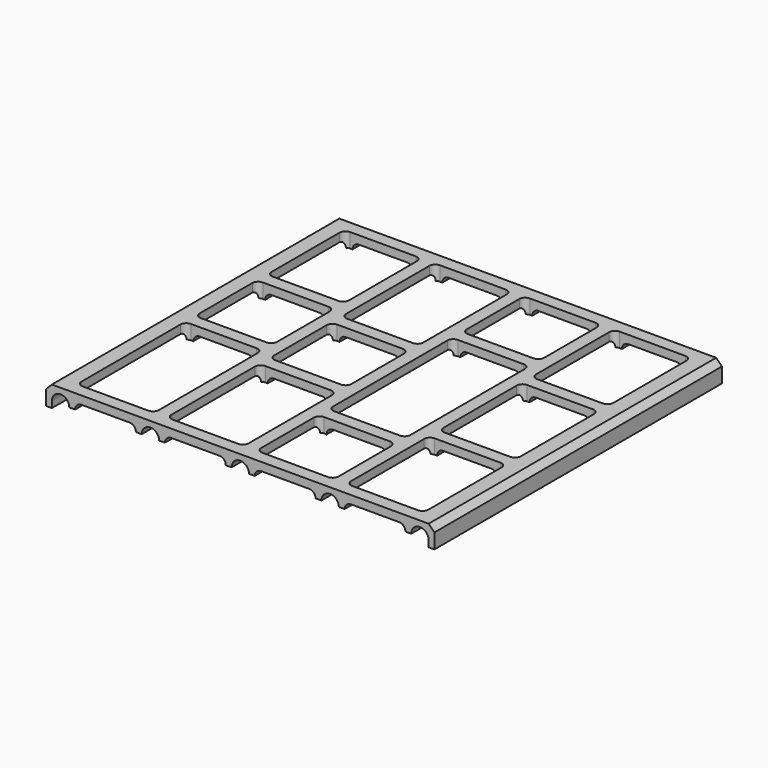
from build123d import *

# Parameters (mm, degrees)
F2_DEPTH      = 74.4
F3_R          = 1.29999
F4_SIZE       = 1.2
F6_W          = 16
F6_H          = 20
F6_H_2        = 16
F6_H_3        = 28
F6_H_4        = 24
F6_H_5        = 32
F6_H_6        = 21.3333333333
F7_DEPTH      = 1.701
F7_DEPTH_BACK = 2.601
F8_T4_DEPTH   = 4.7550100402
F8_S6_R       = 1.8
F8_T7_DEPTH   = 4
F8_T11_DEPTH  = 4.7550100402
F8_S12_R      = 1.8
F8_T13_DEPTH  = 4
F8_T18_DEPTH  = 4.7550100402
F8_S19_R      = 1.8
F8_T20_DEPTH  = 4
F8_T25_DEPTH  = 4.7550100402
F8_S26_R      = 1.8
F8_T27_DEPTH  = 4
F8_T32_DEPTH  = 4.7550100402
F8_S33_R      = 1.8
F8_T34_DEPTH  = 4
F8_T39_DEPTH  = 4.7550100402
F8_S40_R      = 1.8
F8_T41_DEPTH  = 4
F8_T46_DEPTH  = 4.7550100402
F8_S47_R      = 1.8
F8_T48_DEPTH  = 4
F8_T53_DEPTH  = 4.7550100402
F8_S54_R      = 1.8
F8_T55_DEPTH  = 4
F8_T60_DEPTH  = 4.7550100402
F8_S61_R      = 1.8
F8_T62_DEPTH  = 4
F8_T67_DEPTH  = 4.7550100402
F8_S68_R      = 1.8
F8_T69_DEPTH  = 4
F8_T74_DEPTH  = 4.7550100402
F8_S75_R      = 1.8
F8_T76_DEPTH  = 4
F8_T81_DEPTH  = 4.7550100402
F8_S82_R      = 1.8
F8_T83_DEPTH  = 4
F8_T88_DEPTH  = 4.7550100402
F8_S89_R      = 1.8
F8_T90_DEPTH  = 4
F8_T95_DEPTH  = 4.7550100402
F8_S96_R      = 1.8
F8_T97_DEPTH  = 4
F8_T102_DEPTH = 4.7550100402
F8_S103_R     = 1.8
F8_T104_DEPTH = 4
F8_T109_DEPTH = 4.7550100402
F8_S110_R     = 1.8
F8_T111_DEPTH = 4
F8_T116_DEPTH = 4.7550100402
F8_S117_R     = 1.8
F8_T118_DEPTH = 4
F8_T123_DEPTH = 4.7550100402
F8_S125_R     = 1.8
F8_T126_DEPTH = 4
F8_T130_DEPTH = 4.7550100402
F8_S131_R     = 1.8
F8_T132_DEPTH = 4
F8_T137_DEPTH = 4.7550100402
F8_S138_R     = 1.8
F8_T139_DEPTH = 4
F8_T144_DEPTH = 4.7550100402
F8_S145_R     = 1.8
F8_T146_DEPTH = 4
F8_T151_DEPTH = 4.7550100402
F8_S152_R     = 1.8
F8_T153_DEPTH = 4
F8_T158_DEPTH = 4.7550100402
F8_S159_R     = 1.8
F8_T160_DEPTH = 4
F8_T165_DEPTH = 4.7550100402
F8_S166_R     = 1.8
F8_T167_DEPTH = 4
F8_T172_DEPTH = 4.7550100402
F8_S173_R     = 1.8
F8_T174_DEPTH = 4
F8_T179_DEPTH = 4.7550100402
F8_S180_R     = 1.8
F8_T181_DEPTH = 4
F8_T186_DEPTH = 4.7550100402
F8_S187_R     = 1.8
F8_T188_DEPTH = 4
F8_T193_DEPTH = 4.7550100402
F8_S194_R     = 1.8
F8_T195_DEPTH = 4
F8_T200_DEPTH = 4.7550100402
F8_S201_R     = 1.8
F8_T202_DEPTH = 4
F8_T207_DEPTH = 4.7550100402
F8_S209_R     = 1.8
F8_T210_DEPTH = 4
F8_T214_DEPTH = 4.7550100402
F8_S216_R     = 1.8
F8_T217_DEPTH = 4
F8_T221_DEPTH = 4.7550100402
F8_S222_R     = 1.8
F8_T223_DEPTH = 4
F8_T228_DEPTH = 4.7550100402
F8_S229_R     = 1.8
F8_T230_DEPTH = 4
F8_T235_DEPTH = 4.7550100402
F8_S236_R     = 1.8
F8_T237_DEPTH = 4
F8_T242_DEPTH = 4.7550100402
F8_S243_R     = 1.8
F8_T244_DEPTH = 4
F8_T249_DEPTH = 4.7550100402
F8_S250_R     = 1.8
F8_T251_DEPTH = 4
F8_T256_DEPTH = 4.7550100402
F8_S257_R     = 1.8
F8_T258_DEPTH = 4
F8_T263_DEPTH = 4.7550100402
F8_S264_R     = 1.8
F8_T265_DEPTH = 4
F8_T270_DEPTH = 4.7550100402
F8_S271_R     = 1.8
F8_T272_DEPTH = 4
F8_T277_DEPTH = 4.7550100402
F8_S278_R     = 1.8
F8_T279_DEPTH = 4
F8_T284_DEPTH = 4.7550100402
F8_S285_R     = 1.8
F8_T286_DEPTH = 4
F8_T291_DEPTH = 4.7550100402
F8_S292_R     = 1.8
F8_T293_DEPTH = 4
F8_T298_DEPTH = 4.7550100402
F8_S299_R     = 1.8
F8_T300_DEPTH = 4
F8_T305_DEPTH = 4.7550100402
F8_S306_R     = 1.8
F8_T307_DEPTH = 4
F8_T312_DEPTH = 4.7550100402
F8_S313_R     = 1.8
F8_T314_DEPTH = 4
F8_T319_DEPTH = 4.7550100402
F8_S320_R     = 1.8
F8_T321_DEPTH = 4
F8_T326_DEPTH = 4.7550100402
F8_S327_R     = 1.8
F8_T328_DEPTH = 4
F8_T333_DEPTH = 4.7550100402
F8_S334_R     = 1.8
F8_T335_DEPTH = 4


# Not quite as in the source:
# - a fillet or chamfer that OpenCascade refuses, or shapes differently, is made with other operations: its cross-section is extruded or revolved along the edge and cut away or added
# - a fillet or chamfer is up to 0.001 mm smaller than in the source, because OpenCascade refuses the exact size


with BuildPart() as f2:
    # F1 (on Front) → F2 (new body)
    with BuildSketch(Plane.XZ):
        with BuildLine():
            ThreePointArc((-39, -1.3), (-37.2, 0.5), (-35.4, -1.3))
            Line((-35.4, -1.3), (-34.2, -1.3))
            Line((-34.2, -1.3), (-34.2, 0))
            Line((-34.2, 0), (-21.6, 0))
            Line((-21.6, 0), (-21.6, -1.3))
            Line((-21.6, -1.3), (-20.4, -1.3))
            ThreePointArc((-20.4, -1.3), (-18.6, 0.5), (-16.8, -1.3))
            Line((-16.8, -1.3), (-15.6, -1.3))
            Line((-15.6, -1.3), (-15.6, 0))
            Line((-15.6, 0), (-3, 0))
            Line((-3, 0), (-3, -1.3))
            Line((-3, -1.3), (-1.8, -1.3))
            ThreePointArc((-1.8, -1.3), (-1.2727922061, -0.0272077939), (0, 0.5))
            Line((0, 0.5), (0, 1.7))
            Line((0, 1.7), (-40.2, 1.7))
            Line((-40.2, 1.7), (-40.2, -2.6))
            Line((-40.2, -2.6), (-39, -2.6))
            Line((-39, -2.6), (-39, -1.3))
        make_face()
    extrude(amount=F2_DEPTH)

    # F3 (radius 1.3 in the source; OpenCascade refuses exactly that, so slightly less here)
    f3_edges = [f2.edges().sort_by_distance(p)[0] for p in [
        (-34.2, -37.2, 0),
        (-21.6, -37.2, 0),
        (-15.6, -37.2, 0),
        (-3, -37.2, 0),
    ]]
    fillet(f3_edges, radius=F3_R)

    # F4
    f4_edges = [f2.edges().sort_by_distance(p)[0] for p in [
        (-40.2, -37.2, 1.7),
    ]]
    chamfer(f4_edges, length=F4_SIZE)

    # F5: F2 across plane


with BuildPart() as f2_1:
    add(f2.part)
    add(f2.part.mirror(Plane.YZ))

    # F6 (on Top) → F7 (cut, two sides)
    with BuildSketch(Plane.XY) as f7_sk:
        with Locations((-27.9, -12.6)):
            Rectangle(F6_W, F6_H)
        with Locations((-27.9, -33.2)):
            Rectangle(F6_W, F6_H_2)
        with Locations((-27.9, -57.8)):
            Rectangle(F6_W, F6_H_3)
        with Locations((-9.3, -59.8)):
            Rectangle(F6_W, F6_H_4)
        with Locations((9.3, -63.8)):
            Rectangle(F6_W, F6_H_2)
        with Locations((-9.3, -37.2)):
            Rectangle(F6_W, F6_H_2)
        with Locations((-9.3, -14.6)):
            Rectangle(F6_W, F6_H_4)
        with Locations((9.3, -10.6)):
            Rectangle(F6_W, F6_H_2)
        with Locations((9.3, -37.2)):
            Rectangle(F6_W, F6_H_5)
        with Locations((27.9, -13.2666666667)):
            Rectangle(F6_W, F6_H_6)
        with Locations((27.9, -61.1333333333)):
            Rectangle(F6_W, F6_H_6)
        with Locations((27.9, -37.2)):
            Rectangle(F6_W, F6_H_6)
    extrude(amount=F7_DEPTH, mode=Mode.SUBTRACT)
    extrude(f7_sk.sketch, amount=-F7_DEPTH_BACK, mode=Mode.SUBTRACT)

    # F8: fillet of radius 1.2 on 48 edges, made by hand


with BuildPart() as f8_tool2:
    # F8_s3 → F8_t4 (new body)
    with BuildSketch(Plane.XY.offset(1.7)):
        with BuildLine():
            ThreePointArc((-21.1, -2.6), (-20.2514718626, -2.9514718626), (-19.9, -3.8))
            Line((-19.9, -3.8), (-19.9, -2.6))
            Line((-19.9, -2.6), (-21.1, -2.6))
        make_face()
    extrude(amount=-F8_T4_DEPTH)

    split(bisect_by=Plane.XY.offset(-1.3), keep=Keep.TOP)

    # F8_s6 → F8_t7 (cut, symmetric)
    with BuildSketch(Plane.XZ.offset(3.2)):
        with Locations((-18.6, -1.3)):
            Circle(F8_S6_R)
    extrude(amount=F8_T7_DEPTH, both=True, mode=Mode.SUBTRACT)


with BuildPart() as f2_2:
    add(f2_1.part)

    # F8_t1: union F8_tool2
    add(f8_tool2.part)


with BuildPart() as f8_tool9:
    # F8_s10 → F8_t11 (new body)
    with BuildSketch(Plane.XY.offset(-3.0550100402)):
        with BuildLine():
            ThreePointArc((-34.7, -2.6), (-35.5485281374, -2.9514718626), (-35.9, -3.8))
            Line((-35.9, -3.8), (-35.9, -2.6))
            Line((-35.9, -2.6), (-34.7, -2.6))
        make_face()
    extrude(amount=F8_T11_DEPTH)

    # F8_s12 → F8_t13 (cut, symmetric)
    with BuildSketch(Plane.XZ.offset(3.2)):
        with Locations((-37.2, -1.3)):
            Circle(F8_S12_R)
    extrude(amount=F8_T13_DEPTH, both=True, mode=Mode.SUBTRACT)

    split(bisect_by=Plane.XY.offset(-1.3), keep=Keep.TOP)


with BuildPart() as f2_3:
    add(f2_2.part)

    # F8_t8: union F8_tool9
    add(f8_tool9.part)


with BuildPart() as f8_tool16:
    # F8_s17 → F8_t18 (new body)
    with BuildSketch(Plane.XY.offset(1.7)):
        with BuildLine():
            ThreePointArc((-21.1, -22.6), (-20.2514718626, -22.2485281374), (-19.9, -21.4))
            Line((-19.9, -21.4), (-19.9, -22.6))
            Line((-19.9, -22.6), (-21.1, -22.6))
        make_face()
    extrude(amount=-F8_T18_DEPTH)

    # F8_s19 → F8_t20 (cut, symmetric)
    with BuildSketch(Plane.XZ.offset(22)):
        with Locations((-18.6, -1.3)):
            Circle(F8_S19_R)
    extrude(amount=F8_T20_DEPTH, both=True, mode=Mode.SUBTRACT)

    split(bisect_by=Plane.XY.offset(-1.3), keep=Keep.TOP)


with BuildPart() as f2_4:
    add(f2_3.part)

    # F8_t15: union F8_tool16
    add(f8_tool16.part)


with BuildPart() as f8_tool23:
    # F8_s24 → F8_t25 (new body)
    with BuildSketch(Plane.XY.offset(-3.0550100402)):
        with BuildLine():
            ThreePointArc((-35.9, -21.4), (-35.5485281374, -22.2485281374), (-34.7, -22.6))
            Line((-34.7, -22.6), (-35.9, -22.6))
            Line((-35.9, -22.6), (-35.9, -21.4))
        make_face()
    extrude(amount=F8_T25_DEPTH)

    # F8_s26 → F8_t27 (cut, symmetric)
    with BuildSketch(Plane.XZ.offset(22)):
        with Locations((-37.2, -1.3)):
            Circle(F8_S26_R)
    extrude(amount=F8_T27_DEPTH, both=True, mode=Mode.SUBTRACT)

    split(bisect_by=Plane.XY.offset(-1.3), keep=Keep.TOP)


with BuildPart() as f2_5:
    add(f2_4.part)

    # F8_t22: union F8_tool23
    add(f8_tool23.part)


with BuildPart() as f8_tool30:
    # F8_s31 → F8_t32 (new body)
    with BuildSketch(Plane.XY.offset(-3.0550100402)):
        with BuildLine():
            ThreePointArc((-34.7, -25.2), (-35.5485281374, -25.5514718626), (-35.9, -26.4))
            Line((-35.9, -26.4), (-35.9, -25.2))
            Line((-35.9, -25.2), (-34.7, -25.2))
        make_face()
    extrude(amount=F8_T32_DEPTH)

    # F8_s33 → F8_t34 (cut, symmetric)
    with BuildSketch(Plane.XZ.offset(25.8)):
        with Locations((-37.2, -1.3)):
            Circle(F8_S33_R)
    extrude(amount=F8_T34_DEPTH, both=True, mode=Mode.SUBTRACT)

    split(bisect_by=Plane.XY.offset(-1.3), keep=Keep.TOP)


with BuildPart() as f2_6:
    add(f2_5.part)

    # F8_t29: union F8_tool30
    add(f8_tool30.part)


with BuildPart() as f8_tool37:
    # F8_s38 → F8_t39 (new body)
    with BuildSketch(Plane.XY.offset(-3.0550100402)):
        with BuildLine():
            ThreePointArc((-35.9, -40), (-35.5485281374, -40.8485281374), (-34.7, -41.2))
            Line((-34.7, -41.2), (-35.9, -41.2))
            Line((-35.9, -41.2), (-35.9, -40))
        make_face()
    extrude(amount=F8_T39_DEPTH)

    # F8_s40 → F8_t41 (cut, symmetric)
    with BuildSketch(Plane.XZ.offset(40.6)):
        with Locations((-37.2, -1.3)):
            Circle(F8_S40_R)
    extrude(amount=F8_T41_DEPTH, both=True, mode=Mode.SUBTRACT)

    split(bisect_by=Plane.XY.offset(-1.3), keep=Keep.TOP)


with BuildPart() as f2_7:
    add(f2_6.part)

    # F8_t36: union F8_tool37
    add(f8_tool37.part)


with BuildPart() as f8_tool44:
    # F8_s45 → F8_t46 (new body)
    with BuildSketch(Plane.XY.offset(-3.0550100402)):
        with BuildLine():
            ThreePointArc((-35.9, -70.6), (-35.5485281374, -71.4485281374), (-34.7, -71.8))
            Line((-34.7, -71.8), (-35.9, -71.8))
            Line((-35.9, -71.8), (-35.9, -70.6))
        make_face()
    extrude(amount=F8_T46_DEPTH)

    # F8_s47 → F8_t48 (cut, symmetric)
    with BuildSketch(Plane.XZ.offset(71.2)):
        with Locations((-37.2, -1.3)):
            Circle(F8_S47_R)
    extrude(amount=F8_T48_DEPTH, both=True, mode=Mode.SUBTRACT)

    split(bisect_by=Plane.XY.offset(-1.3), keep=Keep.TOP)


with BuildPart() as f2_8:
    add(f2_7.part)

    # F8_t43: union F8_tool44
    add(f8_tool44.part)


with BuildPart() as f8_tool51:
    # F8_s52 → F8_t53 (new body)
    with BuildSketch(Plane.XY.offset(-3.0550100402)):
        with BuildLine():
            ThreePointArc((-34.7, -43.8), (-35.5485281374, -44.1514718626), (-35.9, -45))
            Line((-35.9, -45), (-35.9, -43.8))
            Line((-35.9, -43.8), (-34.7, -43.8))
        make_face()
    extrude(amount=F8_T53_DEPTH)

    # F8_s54 → F8_t55 (cut, symmetric)
    with BuildSketch(Plane.XZ.offset(44.4)):
        with Locations((-37.2, -1.3)):
            Circle(F8_S54_R)
    extrude(amount=F8_T55_DEPTH, both=True, mode=Mode.SUBTRACT)

    split(bisect_by=Plane.XY.offset(-1.3), keep=Keep.TOP)


with BuildPart() as f2_9:
    add(f2_8.part)

    # F8_t50: union F8_tool51
    add(f8_tool51.part)


with BuildPart() as f8_tool58:
    # F8_s59 → F8_t60 (new body)
    with BuildSketch(Plane.XY.offset(1.7)):
        with BuildLine():
            ThreePointArc((-21.1, -25.2), (-20.2514718626, -25.5514718626), (-19.9, -26.4))
            Line((-19.9, -26.4), (-19.9, -25.2))
            Line((-19.9, -25.2), (-21.1, -25.2))
        make_face()
    extrude(amount=-F8_T60_DEPTH)

    # F8_s61 → F8_t62 (cut, symmetric)
    with BuildSketch(Plane.XZ.offset(25.8)):
        with Locations((-18.6, -1.3)):
            Circle(F8_S61_R)
    extrude(amount=F8_T62_DEPTH, both=True, mode=Mode.SUBTRACT)

    split(bisect_by=Plane.XY.offset(-1.3), keep=Keep.TOP)


with BuildPart() as f2_10:
    add(f2_9.part)

    # F8_t57: union F8_tool58
    add(f8_tool58.part)


with BuildPart() as f8_tool65:
    # F8_s66 → F8_t67 (new body)
    with BuildSketch(Plane.XY.offset(1.7)):
        with BuildLine():
            ThreePointArc((-21.1, -41.2), (-20.2514718626, -40.8485281374), (-19.9, -40))
            Line((-19.9, -40), (-19.9, -41.2))
            Line((-19.9, -41.2), (-21.1, -41.2))
        make_face()
    extrude(amount=-F8_T67_DEPTH)

    # F8_s68 → F8_t69 (cut, symmetric)
    with BuildSketch(Plane.XZ.offset(40.6)):
        with Locations((-18.6, -1.3)):
            Circle(F8_S68_R)
    extrude(amount=F8_T69_DEPTH, both=True, mode=Mode.SUBTRACT)

    split(bisect_by=Plane.XY.offset(-1.3), keep=Keep.TOP)


with BuildPart() as f2_11:
    add(f2_10.part)

    # F8_t64: union F8_tool65
    add(f8_tool65.part)


with BuildPart() as f8_tool72:
    # F8_s73 → F8_t74 (new body)
    with BuildSketch(Plane.XY.offset(1.7)):
        with BuildLine():
            ThreePointArc((-21.1, -43.8), (-20.2514718626, -44.1514718626), (-19.9, -45))
            Line((-19.9, -45), (-19.9, -43.8))
            Line((-19.9, -43.8), (-21.1, -43.8))
        make_face()
    extrude(amount=-F8_T74_DEPTH)

    # F8_s75 → F8_t76 (cut, symmetric)
    with BuildSketch(Plane.XZ.offset(44.4)):
        with Locations((-18.6, -1.3)):
            Circle(F8_S75_R)
    extrude(amount=F8_T76_DEPTH, both=True, mode=Mode.SUBTRACT)

    split(bisect_by=Plane.XY.offset(-1.3), keep=Keep.TOP)


with BuildPart() as f2_12:
    add(f2_11.part)

    # F8_t71: union F8_tool72
    add(f8_tool72.part)


with BuildPart() as f8_tool79:
    # F8_s80 → F8_t81 (new body)
    with BuildSketch(Plane.XY.offset(1.7)):
        with BuildLine():
            ThreePointArc((-21.1, -71.8), (-20.2514718626, -71.4485281374), (-19.9, -70.6))
            Line((-19.9, -70.6), (-19.9, -71.8))
            Line((-19.9, -71.8), (-21.1, -71.8))
        make_face()
    extrude(amount=-F8_T81_DEPTH)

    # F8_s82 → F8_t83 (cut, symmetric)
    with BuildSketch(Plane.XZ.offset(71.2)):
        with Locations((-18.6, -1.3)):
            Circle(F8_S82_R)
    extrude(amount=F8_T83_DEPTH, both=True, mode=Mode.SUBTRACT)

    split(bisect_by=Plane.XY.offset(-1.3), keep=Keep.TOP)


with BuildPart() as f2_13:
    add(f2_12.part)

    # F8_t78: union F8_tool79
    add(f8_tool79.part)


with BuildPart() as f8_tool86:
    # F8_s87 → F8_t88 (new body)
    with BuildSketch(Plane.XY.offset(-3.0550100402)):
        with BuildLine():
            ThreePointArc((-17.3, -25.4), (-16.9485281374, -26.2485281374), (-16.1, -26.6))
            Line((-16.1, -26.6), (-17.3, -26.6))
            Line((-17.3, -26.6), (-17.3, -25.4))
        make_face()
    extrude(amount=F8_T88_DEPTH)

    # F8_s89 → F8_t90 (cut, symmetric)
    with BuildSketch(Plane.XZ.offset(26)):
        with Locations((-18.6, -1.3)):
            Circle(F8_S89_R)
    extrude(amount=F8_T90_DEPTH, both=True, mode=Mode.SUBTRACT)

    split(bisect_by=Plane.XY.offset(-1.3), keep=Keep.TOP)


with BuildPart() as f2_14:
    add(f2_13.part)

    # F8_t85: union F8_tool86
    add(f8_tool86.part)


with BuildPart() as f8_tool93:
    # F8_s94 → F8_t95 (new body)
    with BuildSketch(Plane.XY.offset(-3.0550100402)):
        with BuildLine():
            ThreePointArc((-17.3, -44), (-16.9485281374, -44.8485281374), (-16.1, -45.2))
            Line((-16.1, -45.2), (-17.3, -45.2))
            Line((-17.3, -45.2), (-17.3, -44))
        make_face()
    extrude(amount=F8_T95_DEPTH)

    # F8_s96 → F8_t97 (cut, symmetric)
    with BuildSketch(Plane.XZ.offset(44.6)):
        with Locations((-18.6, -1.3)):
            Circle(F8_S96_R)
    extrude(amount=F8_T97_DEPTH, both=True, mode=Mode.SUBTRACT)

    split(bisect_by=Plane.XY.offset(-1.3), keep=Keep.TOP)


with BuildPart() as f2_15:
    add(f2_14.part)

    # F8_t92: union F8_tool93
    add(f8_tool93.part)


with BuildPart() as f8_tool100:
    # F8_s101 → F8_t102 (new body)
    with BuildSketch(Plane.XY.offset(-3.0550100402)):
        with BuildLine():
            ThreePointArc((-17.3, -70.6), (-16.9485281374, -71.4485281374), (-16.1, -71.8))
            Line((-16.1, -71.8), (-17.3, -71.8))
            Line((-17.3, -71.8), (-17.3, -70.6))
        make_face()
    extrude(amount=F8_T102_DEPTH)

    # F8_s103 → F8_t104 (cut, symmetric)
    with BuildSketch(Plane.XZ.offset(71.2)):
        with Locations((-18.6, -1.3)):
            Circle(F8_S103_R)
    extrude(amount=F8_T104_DEPTH, both=True, mode=Mode.SUBTRACT)

    split(bisect_by=Plane.XY.offset(-1.3), keep=Keep.TOP)


with BuildPart() as f2_16:
    add(f2_15.part)

    # F8_t99: union F8_tool100
    add(f8_tool100.part)


with BuildPart() as f8_tool107:
    # F8_s108 → F8_t109 (new body)
    with BuildSketch(Plane.XY.offset(-3.0550100402)):
        with BuildLine():
            ThreePointArc((-16.1, -2.6), (-16.9485281374, -2.9514718626), (-17.3, -3.8))
            Line((-17.3, -3.8), (-17.3, -2.6))
            Line((-17.3, -2.6), (-16.1, -2.6))
        make_face()
    extrude(amount=F8_T109_DEPTH)

    # F8_s110 → F8_t111 (cut, symmetric)
    with BuildSketch(Plane.XZ.offset(3.2)):
        with Locations((-18.6, -1.3)):
            Circle(F8_S110_R)
    extrude(amount=F8_T111_DEPTH, both=True, mode=Mode.SUBTRACT)

    split(bisect_by=Plane.XY.offset(-1.3), keep=Keep.TOP)


with BuildPart() as f2_17:
    add(f2_16.part)

    # F8_t106: union F8_tool107
    add(f8_tool107.part)


with BuildPart() as f8_tool114:
    # F8_s115 → F8_t116 (new body)
    with BuildSketch(Plane.XY.offset(-3.0550100402)):
        with BuildLine():
            ThreePointArc((-16.1, -29.2), (-16.9485281374, -29.5514718626), (-17.3, -30.4))
            Line((-17.3, -30.4), (-17.3, -29.2))
            Line((-17.3, -29.2), (-16.1, -29.2))
        make_face()
    extrude(amount=F8_T116_DEPTH)

    # F8_s117 → F8_t118 (cut, symmetric)
    with BuildSketch(Plane.XZ.offset(29.8)):
        with Locations((-18.6, -1.3)):
            Circle(F8_S117_R)
    extrude(amount=F8_T118_DEPTH, both=True, mode=Mode.SUBTRACT)

    split(bisect_by=Plane.XY.offset(-1.3), keep=Keep.TOP)


with BuildPart() as f2_18:
    add(f2_17.part)

    # F8_t113: union F8_tool114
    add(f8_tool114.part)


with BuildPart() as f8_tool121:
    # F8_s122 → F8_t123 (new body)
    with BuildSketch(Plane.XY.offset(1.7)):
        with BuildLine():
            ThreePointArc((-2.5, -2.6), (-1.6514718626, -2.9514718626), (-1.3, -3.8))
            Line((-1.3, -3.8), (-1.3, -2.6))
            Line((-1.3, -2.6), (-2.5, -2.6))
        make_face()
    extrude(amount=-F8_T123_DEPTH)

    split(bisect_by=Plane.XY.offset(-1.3), keep=Keep.TOP)

    # F8_s125 → F8_t126 (cut, symmetric)
    with BuildSketch(Plane.XZ.offset(3.2)):
        with Locations((0, -1.3)):
            Circle(F8_S125_R)
    extrude(amount=F8_T126_DEPTH, both=True, mode=Mode.SUBTRACT)


with BuildPart() as f2_19:
    add(f2_18.part)

    # F8_t120: union F8_tool121
    add(f8_tool121.part)


with BuildPart() as f8_tool128:
    # F8_s129 → F8_t130 (new body)
    with BuildSketch(Plane.XY.offset(1.7)):
        with BuildLine():
            ThreePointArc((-2.5, -29.2), (-1.6514718626, -29.5514718626), (-1.3, -30.4))
            Line((-1.3, -30.4), (-1.3, -29.2))
            Line((-1.3, -29.2), (-2.5, -29.2))
        make_face()
    extrude(amount=-F8_T130_DEPTH)

    # F8_s131 → F8_t132 (cut, symmetric)
    with BuildSketch(Plane.XZ.offset(29.8)):
        with Locations((0, -1.3)):
            Circle(F8_S131_R)
    extrude(amount=F8_T132_DEPTH, both=True, mode=Mode.SUBTRACT)

    split(bisect_by=Plane.XY.offset(-1.3), keep=Keep.TOP)


with BuildPart() as f2_20:
    add(f2_19.part)

    # F8_t127: union F8_tool128
    add(f8_tool128.part)


with BuildPart() as f8_tool135:
    # F8_s136 → F8_t137 (new body)
    with BuildSketch(Plane.XY.offset(1.7)):
        with BuildLine():
            ThreePointArc((-2.5, -47.8), (-1.6514718626, -48.1514718626), (-1.3, -49))
            Line((-1.3, -49), (-1.3, -47.8))
            Line((-1.3, -47.8), (-2.5, -47.8))
        make_face()
    extrude(amount=-F8_T137_DEPTH)

    # F8_s138 → F8_t139 (cut, symmetric)
    with BuildSketch(Plane.XZ.offset(48.4)):
        with Locations((0, -1.3)):
            Circle(F8_S138_R)
    extrude(amount=F8_T139_DEPTH, both=True, mode=Mode.SUBTRACT)

    split(bisect_by=Plane.XY.offset(-1.3), keep=Keep.TOP)


with BuildPart() as f2_21:
    add(f2_20.part)

    # F8_t134: union F8_tool135
    add(f8_tool135.part)


with BuildPart() as f8_tool142:
    # F8_s143 → F8_t144 (new body)
    with BuildSketch(Plane.XY.offset(1.7)):
        with BuildLine():
            ThreePointArc((-2.5, -71.8), (-1.6514718626, -71.4485281374), (-1.3, -70.6))
            Line((-1.3, -70.6), (-1.3, -71.8))
            Line((-1.3, -71.8), (-2.5, -71.8))
        make_face()
    extrude(amount=-F8_T144_DEPTH)

    # F8_s145 → F8_t146 (cut, symmetric)
    with BuildSketch(Plane.XZ.offset(71.2)):
        with Locations((0, -1.3)):
            Circle(F8_S145_R)
    extrude(amount=F8_T146_DEPTH, both=True, mode=Mode.SUBTRACT)

    split(bisect_by=Plane.XY.offset(-1.3), keep=Keep.TOP)


with BuildPart() as f2_22:
    add(f2_21.part)

    # F8_t141: union F8_tool142
    add(f8_tool142.part)


with BuildPart() as f8_tool149:
    # F8_s150 → F8_t151 (new body)
    with BuildSketch(Plane.XY.offset(1.7)):
        with BuildLine():
            ThreePointArc((-2.5, -45.2), (-1.6514718626, -44.8485281374), (-1.3, -44))
            Line((-1.3, -44), (-1.3, -45.2))
            Line((-1.3, -45.2), (-2.5, -45.2))
        make_face()
    extrude(amount=-F8_T151_DEPTH)

    # F8_s152 → F8_t153 (cut, symmetric)
    with BuildSketch(Plane.XZ.offset(44.6)):
        with Locations((0, -1.3)):
            Circle(F8_S152_R)
    extrude(amount=F8_T153_DEPTH, both=True, mode=Mode.SUBTRACT)

    split(bisect_by=Plane.XY.offset(-1.3), keep=Keep.TOP)


with BuildPart() as f2_23:
    add(f2_22.part)

    # F8_t148: union F8_tool149
    add(f8_tool149.part)


with BuildPart() as f8_tool156:
    # F8_s157 → F8_t158 (new body)
    with BuildSketch(Plane.XY.offset(1.7)):
        with BuildLine():
            ThreePointArc((-2.5, -26.6), (-1.6514718626, -26.2485281374), (-1.3, -25.4))
            Line((-1.3, -25.4), (-1.3, -26.6))
            Line((-1.3, -26.6), (-2.5, -26.6))
        make_face()
    extrude(amount=-F8_T158_DEPTH)

    # F8_s159 → F8_t160 (cut, symmetric)
    with BuildSketch(Plane.XZ.offset(26)):
        with Locations((0, -1.3)):
            Circle(F8_S159_R)
    extrude(amount=F8_T160_DEPTH, both=True, mode=Mode.SUBTRACT)

    split(bisect_by=Plane.XY.offset(-1.3), keep=Keep.TOP)


with BuildPart() as f2_24:
    add(f2_23.part)

    # F8_t155: union F8_tool156
    add(f8_tool156.part)


with BuildPart() as f8_tool163:
    # F8_s164 → F8_t165 (new body)
    with BuildSketch(Plane.XY.offset(-3.0550100402)):
        with BuildLine():
            ThreePointArc((16.1, -71.8), (16.9485281374, -71.4485281374), (17.3, -70.6))
            Line((17.3, -70.6), (17.3, -71.8))
            Line((17.3, -71.8), (16.1, -71.8))
        make_face()
    extrude(amount=F8_T165_DEPTH)

    # F8_s166 → F8_t167 (cut, symmetric)
    with BuildSketch(Plane.XZ.offset(71.2)):
        with Locations((18.6, -1.3)):
            Circle(F8_S166_R)
    extrude(amount=F8_T167_DEPTH, both=True, mode=Mode.SUBTRACT)

    split(bisect_by=Plane.XY.offset(-1.3), keep=Keep.TOP)


with BuildPart() as f2_25:
    add(f2_24.part)

    # F8_t162: union F8_tool163
    add(f8_tool163.part)


with BuildPart() as f8_tool170:
    # F8_s171 → F8_t172 (new body)
    with BuildSketch(Plane.XY.offset(1.7)):
        with BuildLine():
            ThreePointArc((16.1, -53.2), (16.9485281374, -52.8485281374), (17.3, -52))
            Line((17.3, -52), (17.3, -53.2))
            Line((17.3, -53.2), (16.1, -53.2))
        make_face()
    extrude(amount=-F8_T172_DEPTH)

    # F8_s173 → F8_t174 (cut, symmetric)
    with BuildSketch(Plane.XZ.offset(52.6)):
        with Locations((18.6, -1.3)):
            Circle(F8_S173_R)
    extrude(amount=F8_T174_DEPTH, both=True, mode=Mode.SUBTRACT)

    split(bisect_by=Plane.XY.offset(-1.3), keep=Keep.TOP)


with BuildPart() as f2_26:
    add(f2_25.part)

    # F8_t169: union F8_tool170
    add(f8_tool170.part)


with BuildPart() as f8_tool177:
    # F8_s178 → F8_t179 (new body)
    with BuildSketch(Plane.XY.offset(1.7)):
        with BuildLine():
            ThreePointArc((16.1, -18.6), (16.9485281374, -18.2485281374), (17.3, -17.4))
            Line((17.3, -17.4), (17.3, -18.6))
            Line((17.3, -18.6), (16.1, -18.6))
        make_face()
    extrude(amount=-F8_T179_DEPTH)

    # F8_s180 → F8_t181 (cut, symmetric)
    with BuildSketch(Plane.XZ.offset(18)):
        with Locations((18.6, -1.3)):
            Circle(F8_S180_R)
    extrude(amount=F8_T181_DEPTH, both=True, mode=Mode.SUBTRACT)

    split(bisect_by=Plane.XY.offset(-1.3), keep=Keep.TOP)


with BuildPart() as f2_27:
    add(f2_26.part)

    # F8_t176: union F8_tool177
    add(f8_tool177.part)


with BuildPart() as f8_tool184:
    # F8_s185 → F8_t186 (new body)
    with BuildSketch(Plane.XY.offset(1.7)):
        with BuildLine():
            ThreePointArc((34.7, -23.9333333333), (35.5485281374, -23.5818614708), (35.9, -22.7333333333))
            Line((35.9, -22.7333333333), (35.9, -23.9333333333))
            Line((35.9, -23.9333333333), (34.7, -23.9333333333))
        make_face()
    extrude(amount=-F8_T186_DEPTH)

    # F8_s187 → F8_t188 (cut, symmetric)
    with BuildSketch(Plane.XZ.offset(23.3)):
        with Locations((37.2, -1.3)):
            Circle(F8_S187_R)
    extrude(amount=F8_T188_DEPTH, both=True, mode=Mode.SUBTRACT)

    split(bisect_by=Plane.XY.offset(-1.3), keep=Keep.TOP)


with BuildPart() as f2_28:
    add(f2_27.part)

    # F8_t183: union F8_tool184
    add(f8_tool184.part)


with BuildPart() as f8_tool191:
    # F8_s192 → F8_t193 (new body)
    with BuildSketch(Plane.XY.offset(1.7)):
        with BuildLine():
            ThreePointArc((34.7, -47.8666666667), (35.5485281374, -47.5151948041), (35.9, -46.6666666667))
            Line((35.9, -46.6666666667), (35.9, -47.8666666667))
            Line((35.9, -47.8666666667), (34.7, -47.8666666667))
        make_face()
    extrude(amount=-F8_T193_DEPTH)

    # F8_s194 → F8_t195 (cut, symmetric)
    with BuildSketch(Plane.XZ.offset(47.3)):
        with Locations((37.2, -1.3)):
            Circle(F8_S194_R)
    extrude(amount=F8_T195_DEPTH, both=True, mode=Mode.SUBTRACT)

    split(bisect_by=Plane.XY.offset(-1.3), keep=Keep.TOP)


with BuildPart() as f2_29:
    add(f2_28.part)

    # F8_t190: union F8_tool191
    add(f8_tool191.part)


with BuildPart() as f8_tool198:
    # F8_s199 → F8_t200 (new body)
    with BuildSketch(Plane.XY.offset(-3.0550100402)):
        with BuildLine():
            ThreePointArc((34.7, -71.8), (35.5485281374, -71.4485281374), (35.9, -70.6))
            Line((35.9, -70.6), (35.9, -71.8))
            Line((35.9, -71.8), (34.7, -71.8))
        make_face()
    extrude(amount=F8_T200_DEPTH)

    # F8_s201 → F8_t202 (cut, symmetric)
    with BuildSketch(Plane.XZ.offset(71.2)):
        with Locations((37.2, -1.3)):
            Circle(F8_S201_R)
    extrude(amount=F8_T202_DEPTH, both=True, mode=Mode.SUBTRACT)

    split(bisect_by=Plane.XY.offset(-1.3), keep=Keep.TOP)


with BuildPart() as f2_30:
    add(f2_29.part)

    # F8_t197: union F8_tool198
    add(f8_tool198.part)


with BuildPart() as f8_tool205:
    # F8_s206 → F8_t207 (new body)
    with BuildSketch(Plane.XY.offset(1.7)):
        with BuildLine():
            ThreePointArc((34.7, -2.6), (35.5485281374, -2.9514718626), (35.9, -3.8))
            Line((35.9, -3.8), (35.9, -2.6))
            Line((35.9, -2.6), (34.7, -2.6))
        make_face()
    extrude(amount=-F8_T207_DEPTH)

    split(bisect_by=Plane.XY.offset(-1.3), keep=Keep.TOP)

    # F8_s209 → F8_t210 (cut, symmetric)
    with BuildSketch(Plane.XZ.offset(3.2)):
        with Locations((37.2, -1.3)):
            Circle(F8_S209_R)
    extrude(amount=F8_T210_DEPTH, both=True, mode=Mode.SUBTRACT)


with BuildPart() as f2_31:
    add(f2_30.part)

    # F8_t204: union F8_tool205
    add(f8_tool205.part)


with BuildPart() as f8_tool212:
    # F8_s213 → F8_t214 (new body)
    with BuildSketch(Plane.XY.offset(1.7)):
        with BuildLine():
            ThreePointArc((16.1, -2.6), (16.9485281374, -2.9514718626), (17.3, -3.8))
            Line((17.3, -3.8), (17.3, -2.6))
            Line((17.3, -2.6), (16.1, -2.6))
        make_face()
    extrude(amount=-F8_T214_DEPTH)

    split(bisect_by=Plane.XY.offset(-1.3), keep=Keep.TOP)

    # F8_s216 → F8_t217 (cut, symmetric)
    with BuildSketch(Plane.XZ.offset(3.2)):
        with Locations((18.6, -1.3)):
            Circle(F8_S216_R)
    extrude(amount=F8_T217_DEPTH, both=True, mode=Mode.SUBTRACT)


with BuildPart() as f2_32:
    add(f2_31.part)

    # F8_t211: union F8_tool212
    add(f8_tool212.part)


with BuildPart() as f8_tool219:
    # F8_s220 → F8_t221 (new body)
    with BuildSketch(Plane.XY.offset(1.7)):
        with BuildLine():
            ThreePointArc((16.1, -21.2), (16.9485281374, -21.5514718626), (17.3, -22.4))
            Line((17.3, -22.4), (17.3, -21.2))
            Line((17.3, -21.2), (16.1, -21.2))
        make_face()
    extrude(amount=-F8_T221_DEPTH)

    # F8_s222 → F8_t223 (cut, symmetric)
    with BuildSketch(Plane.XZ.offset(21.8)):
        with Locations((18.6, -1.3)):
            Circle(F8_S222_R)
    extrude(amount=F8_T223_DEPTH, both=True, mode=Mode.SUBTRACT)

    split(bisect_by=Plane.XY.offset(-1.3), keep=Keep.TOP)


with BuildPart() as f2_33:
    add(f2_32.part)

    # F8_t218: union F8_tool219
    add(f8_tool219.part)


with BuildPart() as f8_tool226:
    # F8_s227 → F8_t228 (new body)
    with BuildSketch(Plane.XY.offset(1.7)):
        with BuildLine():
            ThreePointArc((16.1, -55.8), (16.9485281374, -56.1514718626), (17.3, -57))
            Line((17.3, -57), (17.3, -55.8))
            Line((17.3, -55.8), (16.1, -55.8))
        make_face()
    extrude(amount=-F8_T228_DEPTH)

    # F8_s229 → F8_t230 (cut, symmetric)
    with BuildSketch(Plane.XZ.offset(56.4)):
        with Locations((18.6, -1.3)):
            Circle(F8_S229_R)
    extrude(amount=F8_T230_DEPTH, both=True, mode=Mode.SUBTRACT)

    split(bisect_by=Plane.XY.offset(-1.3), keep=Keep.TOP)


with BuildPart() as f2_34:
    add(f2_33.part)

    # F8_t225: union F8_tool226
    add(f8_tool226.part)


with BuildPart() as f8_tool233:
    # F8_s234 → F8_t235 (new body)
    with BuildSketch(Plane.XY.offset(-3.0550100402)):
        with BuildLine():
            ThreePointArc((21.1, -71.8), (20.2514718626, -71.4485281374), (19.9, -70.6))
            Line((19.9, -70.6), (19.9, -71.8))
            Line((19.9, -71.8), (21.1, -71.8))
        make_face()
    extrude(amount=F8_T235_DEPTH)

    # F8_s236 → F8_t237 (cut, symmetric)
    with BuildSketch(Plane.XZ.offset(71.2)):
        with Locations((18.6, -1.3)):
            Circle(F8_S236_R)
    extrude(amount=F8_T237_DEPTH, both=True, mode=Mode.SUBTRACT)

    split(bisect_by=Plane.XY.offset(-1.3), keep=Keep.TOP)


with BuildPart() as f2_35:
    add(f2_34.part)

    # F8_t232: union F8_tool233
    add(f8_tool233.part)


with BuildPart() as f8_tool240:
    # F8_s241 → F8_t242 (new body)
    with BuildSketch(Plane.XY.offset(-3.0550100402)):
        with BuildLine():
            ThreePointArc((1.3, -70.6), (1.6514718626, -71.4485281374), (2.5, -71.8))
            Line((2.5, -71.8), (1.3, -71.8))
            Line((1.3, -71.8), (1.3, -70.6))
        make_face()
    extrude(amount=F8_T242_DEPTH)

    # F8_s243 → F8_t244 (cut, symmetric)
    with BuildSketch(Plane.XZ.offset(71.2)):
        with Locations((0, -1.3)):
            Circle(F8_S243_R)
    extrude(amount=F8_T244_DEPTH, both=True, mode=Mode.SUBTRACT)

    split(bisect_by=Plane.XY.offset(-1.3), keep=Keep.TOP)


with BuildPart() as f2_36:
    add(f2_35.part)

    # F8_t239: union F8_tool240
    add(f8_tool240.part)


with BuildPart() as f8_tool247:
    # F8_s248 → F8_t249 (new body)
    with BuildSketch(Plane.XY.offset(-3.0550100402)):
        with BuildLine():
            ThreePointArc((1.3, -52), (1.6514718626, -52.8485281374), (2.5, -53.2))
            Line((2.5, -53.2), (1.3, -53.2))
            Line((1.3, -53.2), (1.3, -52))
        make_face()
    extrude(amount=F8_T249_DEPTH)

    # F8_s250 → F8_t251 (cut, symmetric)
    with BuildSketch(Plane.XZ.offset(52.6)):
        with Locations((0, -1.3)):
            Circle(F8_S250_R)
    extrude(amount=F8_T251_DEPTH, both=True, mode=Mode.SUBTRACT)

    split(bisect_by=Plane.XY.offset(-1.3), keep=Keep.TOP)


with BuildPart() as f2_37:
    add(f2_36.part)

    # F8_t246: union F8_tool247
    add(f8_tool247.part)


with BuildPart() as f8_tool254:
    # F8_s255 → F8_t256 (new body)
    with BuildSketch(Plane.XY.offset(-3.0550100402)):
        with BuildLine():
            ThreePointArc((1.3, -17.4), (1.6514718626, -18.2485281374), (2.5, -18.6))
            Line((2.5, -18.6), (1.3, -18.6))
            Line((1.3, -18.6), (1.3, -17.4))
        make_face()
    extrude(amount=F8_T256_DEPTH)

    # F8_s257 → F8_t258 (cut, symmetric)
    with BuildSketch(Plane.XZ.offset(18)):
        with Locations((0, -1.3)):
            Circle(F8_S257_R)
    extrude(amount=F8_T258_DEPTH, both=True, mode=Mode.SUBTRACT)

    split(bisect_by=Plane.XY.offset(-1.3), keep=Keep.TOP)


with BuildPart() as f2_38:
    add(f2_37.part)

    # F8_t253: union F8_tool254
    add(f8_tool254.part)


with BuildPart() as f8_tool261:
    # F8_s262 → F8_t263 (new body)
    with BuildSketch(Plane.XY.offset(-3.0550100402)):
        with BuildLine():
            ThreePointArc((21.1, -47.8666666667), (20.2514718626, -47.5151948041), (19.9, -46.6666666667))
            Line((19.9, -46.6666666667), (19.9, -47.8666666667))
            Line((19.9, -47.8666666667), (21.1, -47.8666666667))
        make_face()
    extrude(amount=F8_T263_DEPTH)

    # F8_s264 → F8_t265 (cut, symmetric)
    with BuildSketch(Plane.XZ.offset(47.3)):
        with Locations((18.6, -1.3)):
            Circle(F8_S264_R)
    extrude(amount=F8_T265_DEPTH, both=True, mode=Mode.SUBTRACT)

    split(bisect_by=Plane.XY.offset(-1.3), keep=Keep.TOP)


with BuildPart() as f2_39:
    add(f2_38.part)

    # F8_t260: union F8_tool261
    add(f8_tool261.part)


with BuildPart() as f8_tool268:
    # F8_s269 → F8_t270 (new body)
    with BuildSketch(Plane.XY.offset(-3.0550100402)):
        with BuildLine():
            ThreePointArc((21.1, -23.9333333333), (20.2514718626, -23.5818614708), (19.9, -22.7333333333))
            Line((19.9, -22.7333333333), (19.9, -23.9333333333))
            Line((19.9, -23.9333333333), (21.1, -23.9333333333))
        make_face()
    extrude(amount=F8_T270_DEPTH)

    # F8_s271 → F8_t272 (cut, symmetric)
    with BuildSketch(Plane.XZ.offset(23.3)):
        with Locations((18.6, -1.3)):
            Circle(F8_S271_R)
    extrude(amount=F8_T272_DEPTH, both=True, mode=Mode.SUBTRACT)

    split(bisect_by=Plane.XY.offset(-1.3), keep=Keep.TOP)


with BuildPart() as f2_40:
    add(f2_39.part)

    # F8_t267: union F8_tool268
    add(f8_tool268.part)


with BuildPart() as f8_tool275:
    # F8_s276 → F8_t277 (new body)
    with BuildSketch(Plane.XY.offset(1.7)):
        with BuildLine():
            ThreePointArc((2.5, -55.8), (1.6514718626, -56.1514718626), (1.3, -57))
            Line((1.3, -57), (1.3, -55.8))
            Line((1.3, -55.8), (2.5, -55.8))
        make_face()
    extrude(amount=-F8_T277_DEPTH)

    # F8_s278 → F8_t279 (cut, symmetric)
    with BuildSketch(Plane.XZ.offset(56.4)):
        with Locations((0, -1.3)):
            Circle(F8_S278_R)
    extrude(amount=F8_T279_DEPTH, both=True, mode=Mode.SUBTRACT)

    split(bisect_by=Plane.XY.offset(-1.3), keep=Keep.TOP)


with BuildPart() as f2_41:
    add(f2_40.part)

    # F8_t274: union F8_tool275
    add(f8_tool275.part)


with BuildPart() as f8_tool282:
    # F8_s283 → F8_t284 (new body)
    with BuildSketch(Plane.XY.offset(1.7)):
        with BuildLine():
            ThreePointArc((19.9, -51.6666666667), (20.2514718626, -50.8181385292), (21.1, -50.4666666667))
            Line((21.1, -50.4666666667), (19.9, -50.4666666667))
            Line((19.9, -50.4666666667), (19.9, -51.6666666667))
        make_face()
    extrude(amount=-F8_T284_DEPTH)

    # F8_s285 → F8_t286 (cut, symmetric)
    with BuildSketch(Plane.XZ.offset(51.1)):
        with Locations((18.6, -1.3)):
            Circle(F8_S285_R)
    extrude(amount=F8_T286_DEPTH, both=True, mode=Mode.SUBTRACT)

    split(bisect_by=Plane.XY.offset(-1.3), keep=Keep.TOP)


with BuildPart() as f2_42:
    add(f2_41.part)

    # F8_t281: union F8_tool282
    add(f8_tool282.part)


with BuildPart() as f8_tool289:
    # F8_s290 → F8_t291 (new body)
    with BuildSketch(Plane.XY.offset(-3.0550100402)):
        with BuildLine():
            ThreePointArc((2.5, -21.2), (1.6514718626, -21.5514718626), (1.3, -22.4))
            Line((1.3, -22.4), (1.3, -21.2))
            Line((1.3, -21.2), (2.5, -21.2))
        make_face()
    extrude(amount=F8_T291_DEPTH)

    # F8_s292 → F8_t293 (cut, symmetric)
    with BuildSketch(Plane.XZ.offset(21.8)):
        with Locations((0, -1.3)):
            Circle(F8_S292_R)
    extrude(amount=F8_T293_DEPTH, both=True, mode=Mode.SUBTRACT)

    split(bisect_by=Plane.XY.offset(-1.3), keep=Keep.TOP)


with BuildPart() as f2_43:
    add(f2_42.part)

    # F8_t288: union F8_tool289
    add(f8_tool289.part)


with BuildPart() as f8_tool296:
    # F8_s297 → F8_t298 (new body)
    with BuildSketch(Plane.XY.offset(-3.0550100402)):
        with BuildLine():
            ThreePointArc((19.9, -27.7333333333), (20.2514718626, -26.8848051959), (21.1, -26.5333333333))
            Line((21.1, -26.5333333333), (19.9, -26.5333333333))
            Line((19.9, -26.5333333333), (19.9, -27.7333333333))
        make_face()
    extrude(amount=F8_T298_DEPTH)

    # F8_s299 → F8_t300 (cut, symmetric)
    with BuildSketch(Plane.XZ.offset(27.1)):
        with Locations((18.6, -1.3)):
            Circle(F8_S299_R)
    extrude(amount=F8_T300_DEPTH, both=True, mode=Mode.SUBTRACT)

    split(bisect_by=Plane.XY.offset(-1.3), keep=Keep.TOP)


with BuildPart() as f2_44:
    add(f2_43.part)

    # F8_t295: union F8_tool296
    add(f8_tool296.part)


with BuildPart() as f8_tool303:
    # F8_s304 → F8_t305 (new body)
    with BuildSketch(Plane.XY.offset(-3.0550100402)):
        with BuildLine():
            ThreePointArc((2.5, -2.6), (1.6514718626, -2.9514718626), (1.3, -3.8))
            Line((1.3, -3.8), (1.3, -2.6))
            Line((1.3, -2.6), (2.5, -2.6))
        make_face()
    extrude(amount=F8_T305_DEPTH)

    # F8_s306 → F8_t307 (cut, symmetric)
    with BuildSketch(Plane.XZ.offset(3.2)):
        with Locations((0, -1.3)):
            Circle(F8_S306_R)
    extrude(amount=F8_T307_DEPTH, both=True, mode=Mode.SUBTRACT)

    split(bisect_by=Plane.XY.offset(-1.3), keep=Keep.TOP)


with BuildPart() as f2_45:
    add(f2_44.part)

    # F8_t302: union F8_tool303
    add(f8_tool303.part)


with BuildPart() as f8_tool310:
    # F8_s311 → F8_t312 (new body)
    with BuildSketch(Plane.XY.offset(-3.0550100402)):
        with BuildLine():
            ThreePointArc((19.9, -3.8), (20.2514718626, -2.9514718626), (21.1, -2.6))
            Line((21.1, -2.6), (19.9, -2.6))
            Line((19.9, -2.6), (19.9, -3.8))
        make_face()
    extrude(amount=F8_T312_DEPTH)

    # F8_s313 → F8_t314 (cut, symmetric)
    with BuildSketch(Plane.XZ.offset(3.2)):
        with Locations((18.6, -1.3)):
            Circle(F8_S313_R)
    extrude(amount=F8_T314_DEPTH, both=True, mode=Mode.SUBTRACT)

    split(bisect_by=Plane.XY.offset(-1.3), keep=Keep.TOP)


with BuildPart() as f2_46:
    add(f2_45.part)

    # F8_t309: union F8_tool310
    add(f8_tool310.part)


with BuildPart() as f8_tool317:
    # F8_s318 → F8_t319 (new body)
    with BuildSketch(Plane.XY.offset(-3.0550100402)):
        with BuildLine():
            ThreePointArc((-16.1, -47.8), (-16.9485281374, -48.1514718626), (-17.3, -49))
            Line((-17.3, -49), (-17.3, -47.8))
            Line((-17.3, -47.8), (-16.1, -47.8))
        make_face()
    extrude(amount=F8_T319_DEPTH)

    # F8_s320 → F8_t321 (cut, symmetric)
    with BuildSketch(Plane.XZ.offset(48.4)):
        with Locations((-18.6, -1.3)):
            Circle(F8_S320_R)
    extrude(amount=F8_T321_DEPTH, both=True, mode=Mode.SUBTRACT)

    split(bisect_by=Plane.XY.offset(-1.3), keep=Keep.TOP)


with BuildPart() as f2_47:
    add(f2_46.part)

    # F8_t316: union F8_tool317
    add(f8_tool317.part)


with BuildPart() as f8_tool324:
    # F8_s325 → F8_t326 (new body)
    with BuildSketch(Plane.XY.offset(1.7)):
        with BuildLine():
            ThreePointArc((34.7, -50.4666666667), (35.5485281374, -50.8181385292), (35.9, -51.6666666667))
            Line((35.9, -51.6666666667), (35.9, -50.4666666667))
            Line((35.9, -50.4666666667), (34.7, -50.4666666667))
        make_face()
    extrude(amount=-F8_T326_DEPTH)

    # F8_s327 → F8_t328 (cut, symmetric)
    with BuildSketch(Plane.XZ.offset(51.1)):
        with Locations((37.2, -1.3)):
            Circle(F8_S327_R)
    extrude(amount=F8_T328_DEPTH, both=True, mode=Mode.SUBTRACT)

    split(bisect_by=Plane.XY.offset(-1.3), keep=Keep.TOP)


with BuildPart() as f2_48:
    add(f2_47.part)

    # F8_t323: union F8_tool324
    add(f8_tool324.part)


with BuildPart() as f8_tool331:
    # F8_s332 → F8_t333 (new body)
    with BuildSketch(Plane.XY.offset(1.7)):
        with BuildLine():
            ThreePointArc((34.7, -26.5333333333), (35.5485281374, -26.8848051959), (35.9, -27.7333333333))
            Line((35.9, -27.7333333333), (35.9, -26.5333333333))
            Line((35.9, -26.5333333333), (34.7, -26.5333333333))
        make_face()
    extrude(amount=-F8_T333_DEPTH)

    # F8_s334 → F8_t335 (cut, symmetric)
    with BuildSketch(Plane.XZ.offset(27.1)):
        with Locations((37.2, -1.3)):
            Circle(F8_S334_R)
    extrude(amount=F8_T335_DEPTH, both=True, mode=Mode.SUBTRACT)

    split(bisect_by=Plane.XY.offset(-1.3), keep=Keep.TOP)


with BuildPart() as f2_49:
    add(f2_48.part)

    # F8_t330: union F8_tool331
    add(f8_tool331.part)


solid = f2_49.part
